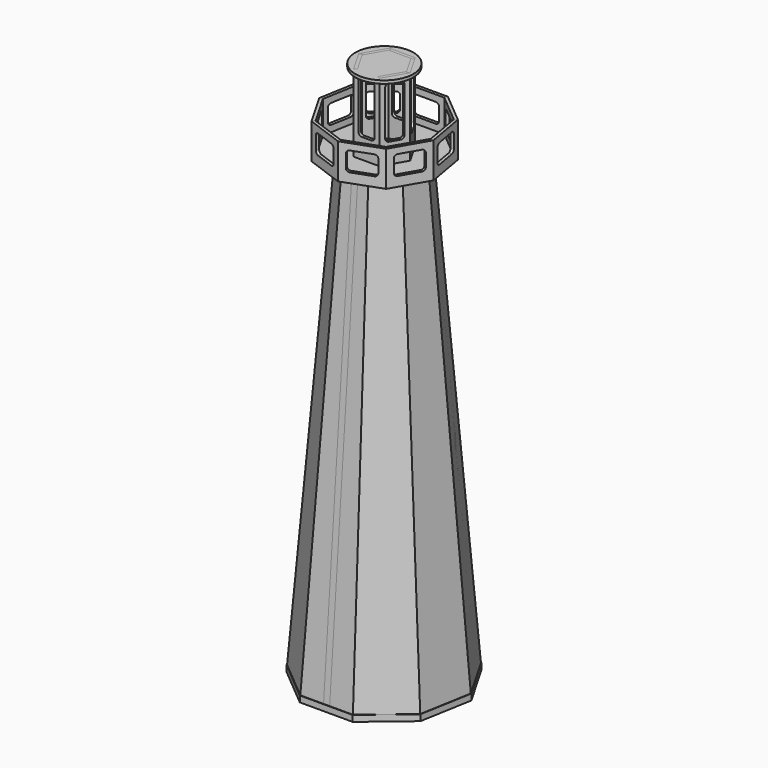
from build123d import *

# Parameters (mm, degrees)
F13_DEPTH = 6
F14_DEPTH = 3
F15_DEPTH = 3
F16_DEPTH = 3
F8_W      = 39.0929023821
F8_H      = 3
F8_H_2    = 31.75
F17_DEPTH = 3
F10_W     = 25.4
F10_H     = 79.2
F18_DEPTH = 3
F12_R     = 28.575
F19_DEPTH = 3
F20_COUNT = 3
F21_COUNT = 9
F22_COUNT = 6


# Not quite as in the source:
# - a feature names something its author has since deleted; it is built from what else it names


with BuildPart() as f13:
    # F1 (on Top) → F13 (new body)
    with BuildSketch(Plane.XY):
        Polygon((48.9804158581, 58.3725865657), (0, 76.2), (-48.9804158581, 58.3725865657), (-75.0423507795, 13.2319911382), (-65.9911357684, -38.1), (-26.0619349214, -71.6045777039), (26.0619349214, -71.6045777039), (65.9911357684, -38.1), (75.0423507795, 13.2319911382), align=None)
    extrude(amount=F13_DEPTH)


with BuildPart() as f14:
    # F5 (on 3pt) → F14 (new body)
    with BuildSketch(Plane(origin=(0, -71.1681674723, 5.5730168174), x_dir=(-1, 0, 0), z_dir=(0, 0.9969479799, -0.0780687217))):
        Polygon((-13.0309674607, 453.0095775028), (-26.0619349214, -5.5900778471), (26.0619349214, -5.5900778471), (13.0309674607, 453.0095775028), align=None)
    extrude(amount=F14_DEPTH)


with BuildPart() as f15:
    # F6 (on Right) → F15 (new body, symmetric)
    with BuildSketch(Plane.YZ):
        Polygon((-16.7522888519, 454.2), (-36.0372120071, 454.2), (-71.6045777039, 0), (-16.7522888519, 0), align=None)
    extrude(amount=F15_DEPTH, both=True)


with BuildPart() as f16:
    # F3 (on offset) → F16 (new body)
    with BuildSketch(Plane.XY.offset(457.2)):
        Polygon((-36.7353118936, -43.7794399242), (0, -57.15), (36.7353118936, -43.7794399242), (56.2817630846, -9.9239933537), (49.4933518263, 28.575), (19.5464511911, 53.7034332779), (-19.5464511911, 53.7034332779), (-49.4933518263, 28.575), (-56.2817630846, -9.9239933537), align=None)
        Polygon((-24.4902079291, 29.1862932828), (0, 38.1), (24.4902079291, 29.1862932828), (37.5211753898, 6.6159955691), (32.9955678842, -19.05), (13.0309674607, -35.8022888519), (-13.0309674607, -35.8022888519), (-32.9955678842, -19.05), (-37.5211753898, 6.6159955691), align=None, mode=Mode.SUBTRACT)
        Polygon((24.4902079291, 29.1862932828), (0, 38.1), (-24.4902079291, 29.1862932828), (-37.5211753898, 6.6159955691), (-32.9955678842, -19.05), (-13.0309674607, -35.8022888519), (13.0309674607, -35.8022888519), (32.9955678842, -19.05), (37.5211753898, 6.6159955691), align=None)
        Polygon((12.7, 21.9970452561), (25.4, 0), (12.7, -21.9970452561), (-12.7, -21.9970452561), (-25.4, 0), (-12.7, 21.9970452561), align=None, mode=Mode.SUBTRACT)
        Polygon((12.7, -21.9970452561), (25.4, 0), (12.7, 21.9970452561), (-12.7, 21.9970452561), (-25.4, 0), (-12.7, -21.9970452561), align=None)
    extrude(amount=-F16_DEPTH)


with BuildPart() as f17:
    # F8 (on plane+point) → F17 (new body)
    with BuildSketch(Plane.XZ.offset(-53.7034332779)):
        with Locations((0, 455.7)):
            Rectangle(F8_W, F8_H)
        with Locations((0, 473.075)):
            Rectangle(F8_W, F8_H_2)
        with BuildLine():
            Line((-10.0214511911, 482.6), (10.0214511911, 482.6))
            ThreePointArc((10.0214511911, 482.6), (12.2665152213, 481.6700640303), (13.1964511911, 479.425))
            Line((13.1964511911, 479.425), (13.1964511911, 466.725))
            ThreePointArc((13.1964511911, 466.725), (12.2665152213, 464.4799359697), (10.0214511911, 463.55))
            Line((10.0214511911, 463.55), (-10.0214511911, 463.55))
            ThreePointArc((-10.0214511911, 463.55), (-12.2665152213, 464.4799359697), (-13.1964511911, 466.725))
            Line((-13.1964511911, 466.725), (-13.1964511911, 479.425))
            ThreePointArc((-13.1964511911, 479.425), (-12.2665152213, 481.6700640303), (-10.0214511911, 482.6))
        make_face(mode=Mode.SUBTRACT)
    extrude(amount=F17_DEPTH)


with BuildPart() as f18:
    # F10 (on plane+point) → F18 (new body)
    with BuildSketch(Plane.XZ.offset(21.9970452561)):
        with Locations((0, 493.8)):
            Rectangle(F10_W, F10_H)
        with BuildLine():
            Line((4.7625, 476.9104), (-4.7625, 476.9104))
            ThreePointArc((-4.7625, 476.9104), (-7.0075640303, 477.8403359697), (-7.9375, 480.0854))
            Line((-7.9375, 480.0854), (-7.9375, 524.5354))
            ThreePointArc((-7.9375, 524.5354), (-7.0075640303, 526.7804640303), (-4.7625, 527.7104))
            Line((-4.7625, 527.7104), (4.7625, 527.7104))
            ThreePointArc((4.7625, 527.7104), (7.0075640303, 526.7804640303), (7.9375, 524.5354))
            Line((7.9375, 524.5354), (7.9375, 480.0854))
            ThreePointArc((7.9375, 480.0854), (7.0075640303, 477.8403359697), (4.7625, 476.9104))
        make_face(mode=Mode.SUBTRACT)
    extrude(amount=-F18_DEPTH)


with BuildPart() as f19:
    # F12 (on plane+point) → F19 (new body)
    with BuildSketch(Plane.XY.offset(533.4)):
        Circle(F12_R)
    extrude(amount=-F19_DEPTH)


with BuildPart() as f20_1:
    # F20: instance of F15
    add(f15.part.rotate(Axis((0, 0, 304.8), (0, 0, 1)), 1 * 360 / F20_COUNT))


with BuildPart() as f20_2:
    # F20: instance of F15
    add(f15.part.rotate(Axis((0, 0, 304.8), (0, 0, 1)), 2 * 360 / F20_COUNT))


with BuildPart() as f21_1:
    # F21: instance of F17
    add(f17.part.rotate(Axis((0, 0, 304.8), (0, 0, 1)), 1 * 360 / F21_COUNT))


with BuildPart() as f21_2:
    # F21: instance of F17
    add(f17.part.rotate(Axis((0, 0, 304.8), (0, 0, 1)), 2 * 360 / F21_COUNT))


with BuildPart() as f21_3:
    # F21: instance of F17
    add(f17.part.rotate(Axis((0, 0, 304.8), (0, 0, 1)), 3 * 360 / F21_COUNT))


with BuildPart() as f21_4:
    # F21: instance of F17
    add(f17.part.rotate(Axis((0, 0, 304.8), (0, 0, 1)), 4 * 360 / F21_COUNT))


with BuildPart() as f21_5:
    # F21: instance of F17
    add(f17.part.rotate(Axis((0, 0, 304.8), (0, 0, 1)), 5 * 360 / F21_COUNT))


with BuildPart() as f21_6:
    # F21: instance of F17
    add(f17.part.rotate(Axis((0, 0, 304.8), (0, 0, 1)), 6 * 360 / F21_COUNT))


with BuildPart() as f21_7:
    # F21: instance of F17
    add(f17.part.rotate(Axis((0, 0, 304.8), (0, 0, 1)), 7 * 360 / F21_COUNT))


with BuildPart() as f21_8:
    # F21: instance of F17
    add(f17.part.rotate(Axis((0, 0, 304.8), (0, 0, 1)), 8 * 360 / F21_COUNT))


with BuildPart() as f21_9:
    # F21: instance of F14
    add(f14.part.rotate(Axis((0, 0, 304.8), (0, 0, 1)), 1 * 360 / F21_COUNT))


with BuildPart() as f21_10:
    # F21: instance of F14
    add(f14.part.rotate(Axis((0, 0, 304.8), (0, 0, 1)), 2 * 360 / F21_COUNT))


with BuildPart() as f21_11:
    # F21: instance of F14
    add(f14.part.rotate(Axis((0, 0, 304.8), (0, 0, 1)), 3 * 360 / F21_COUNT))


with BuildPart() as f21_12:
    # F21: instance of F14
    add(f14.part.rotate(Axis((0, 0, 304.8), (0, 0, 1)), 4 * 360 / F21_COUNT))


with BuildPart() as f21_13:
    # F21: instance of F14
    add(f14.part.rotate(Axis((0, 0, 304.8), (0, 0, 1)), 5 * 360 / F21_COUNT))


with BuildPart() as f21_14:
    # F21: instance of F14
    add(f14.part.rotate(Axis((0, 0, 304.8), (0, 0, 1)), 6 * 360 / F21_COUNT))


with BuildPart() as f21_15:
    # F21: instance of F14
    add(f14.part.rotate(Axis((0, 0, 304.8), (0, 0, 1)), 7 * 360 / F21_COUNT))


with BuildPart() as f21_16:
    # F21: instance of F14
    add(f14.part.rotate(Axis((0, 0, 304.8), (0, 0, 1)), 8 * 360 / F21_COUNT))


with BuildPart() as f22_1:
    # F22: instance of F18
    add(f18.part.rotate(Axis((0, 0, 304.8), (0, 0, 1)), 1 * 360 / F22_COUNT))


with BuildPart() as f22_2:
    # F22: instance of F18
    add(f18.part.rotate(Axis((0, 0, 304.8), (0, 0, 1)), 2 * 360 / F22_COUNT))


with BuildPart() as f22_3:
    # F22: instance of F18
    add(f18.part.rotate(Axis((0, 0, 304.8), (0, 0, 1)), 3 * 360 / F22_COUNT))


with BuildPart() as f22_4:
    # F22: instance of F18
    add(f18.part.rotate(Axis((0, 0, 304.8), (0, 0, 1)), 4 * 360 / F22_COUNT))


with BuildPart() as f22_5:
    # F22: instance of F18
    add(f18.part.rotate(Axis((0, 0, 304.8), (0, 0, 1)), 5 * 360 / F22_COUNT))


solid = Compound([f13.part, f14.part, f15.part, f16.part, f17.part, f18.part, f19.part, f20_1.part, f20_2.part, f21_1.part, f21_2.part, f21_3.part, f21_4.part, f21_5.part, f21_6.part, f21_7.part, f21_8.part, f21_9.part, f21_10.part, f21_11.part, f21_12.part, f21_13.part, f21_14.part, f21_15.part, f21_16.part, f22_1.part, f22_2.part, f22_3.part, f22_4.part, f22_5.part])
